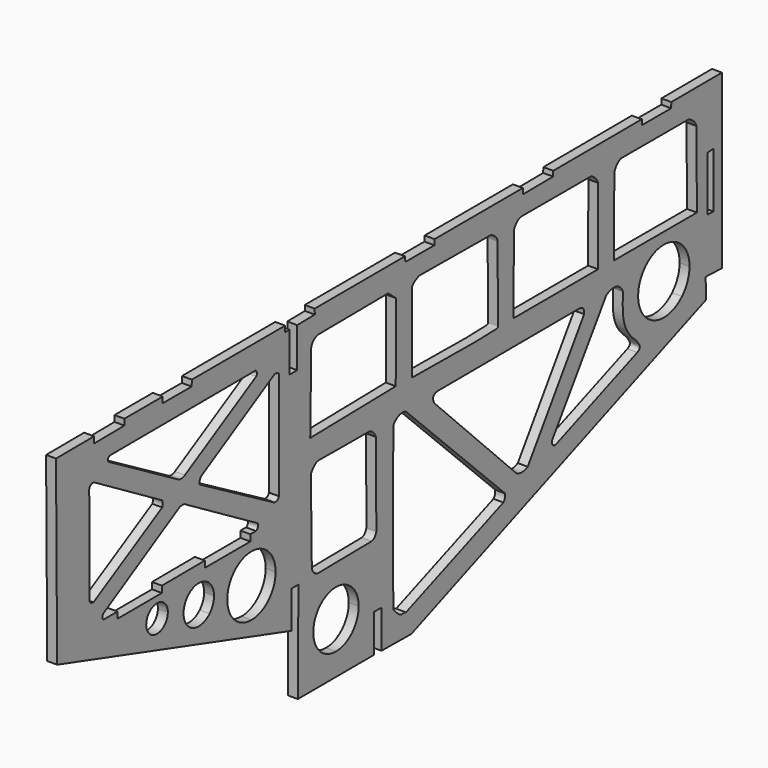
from build123d import *

# Parameters (mm, degrees)
F1_DEPTH = 4


# Not quite as in the source:
# - ends of sketch curves that miss each other by under 0.0002 mm in the source are joined
# - the dataset's text gives a spline's control points without its knots; the knots are read off the source's solid


with BuildPart() as f1:
    # F0 (on Right) → F1 (new body)
    with BuildSketch(Plane.YZ):
        Polygon((-148.644908, 67.35988), (-167.821425, 67.256855), (-167.254463, -6.165021), (-49.042065, -42.167249), (-49.042065, -27.142701), (-45.640268, -27.142701), (-45.92376, -67.680652), (-7.626045, -67.593697), (-7.48542, -52.325631), (-3.764723, -52.349332), (-3.768473, -67.675754), (11.266275, -67.823819), (159.883927, -9.566811), (159.600457, -1.345829), (167.821425, -1.629314), (167.821425, 67.823819), (142.301062, 67.735915), (142.250812, 65.543531), (127.61667, 65.559821), (127.418092, 67.684651), (82.819147, 67.531032), (82.71993, 65.492416), (67.440277, 65.375344), (67.489702, 67.653501), (22.990132, 67.577961), (22.89126, 65.441222), (8.256105, 65.473059), (8.057925, 67.552611), (-37.434053, 67.475386), (-37.384478, 65.338883), (-46.26441, 65.212072), (-46.264583, 49.200648), (-50.03556, 49.197423), (-50.059785, 65.157835), (-52.316775, 65.125607), (-52.316918, 67.503332), (-99.3465, 67.434865), (-99.445935, 65.001045), (-114.179535, 65.035484), (-114.030848, 67.413485), (-133.350465, 67.38536), (-133.37844, 64.951643), (-148.658258, 64.782237), align=None)
        with BuildLine():
            add(Edge.make_bspline(
                [(-18.620168, -39.073955), (-16.475133, -41.218991), (-15.270066, -44.128283), (-15.270067, -47.161822)],
                knots=[0, 0, 0, 0, 1, 1, 1, 1], degree=3))
            add(Edge.make_bspline(
                [(-15.270067, -47.161822), (-15.270069, -53.478835), (-20.391019, -58.599785), (-26.708033, -58.599787)],
                knots=[0, 0, 0, 0, 1, 1, 1, 1], degree=3))
            add(Edge.make_bspline(
                [(-26.708033, -58.599787), (-33.025046, -58.599785), (-38.145996, -53.478835), (-38.145998, -47.161821)],
                knots=[0, 0, 0, 0, 1, 1, 1, 1], degree=3))
            add(Edge.make_bspline(
                [(-38.145998, -47.161821), (-38.145999, -44.128283), (-36.940932, -41.218991), (-34.795897, -39.073955)],
                knots=[0, 0, 0, 0, 1, 1, 1, 1], degree=3))
            add(Edge.make_bspline(
                [(-34.795897, -39.073955), (-32.650862, -36.928919), (-29.741571, -35.72385), (-26.708033, -35.723849)],
                knots=[0, 0, 0, 0, 1, 1, 1, 1], degree=3))
            add(Edge.make_bspline(
                [(-26.708033, -35.723849), (-23.674494, -35.72385), (-20.765203, -36.928919), (-18.620168, -39.073955)],
                knots=[0, 0, 0, 0, 1, 1, 1, 1], degree=3))
        make_face(mode=Mode.SUBTRACT)
        with BuildLine():
            add(Edge.make_bspline(
                [(-116.897902, -4.781812), (-113.891735, -4.781812), (-111.454756, -7.218792), (-111.454755, -10.224959)],
                knots=[0, 0, 0, 0, 1, 1, 1, 1], degree=3))
            add(Edge.make_bspline(
                [(-111.454755, -10.224959), (-111.454756, -13.231126), (-113.891735, -15.668106), (-116.897902, -15.668106)],
                knots=[0, 0, 0, 0, 1, 1, 1, 1], degree=3))
            add(Edge.make_bspline(
                [(-116.897902, -15.668106), (-119.90407, -15.668106), (-122.341049, -13.231126), (-122.34105, -10.224959)],
                knots=[0, 0, 0, 0, 1, 1, 1, 1], degree=3))
            add(Edge.make_bspline(
                [(-122.34105, -10.224959), (-122.341049, -7.218792), (-119.90407, -4.781812), (-116.897902, -4.781812)],
                knots=[0, 0, 0, 0, 1, 1, 1, 1], degree=3))
        make_face(mode=Mode.SUBTRACT)
        with BuildLine():
            add(Edge.make_bspline(
                [(-90.414146, -8.436888), (-88.973656, -9.877378), (-88.164397, -11.831103), (-88.164398, -13.868264)],
                knots=[0, 0, 0, 0, 1, 1, 1, 1], degree=3))
            add(Edge.make_bspline(
                [(-88.164398, -13.868264), (-88.164397, -15.905425), (-88.973656, -17.85915), (-90.414146, -19.29964)],
                knots=[0, 0, 0, 0, 1, 1, 1, 1], degree=3))
            add(Edge.make_bspline(
                [(-90.414146, -19.29964), (-91.854637, -20.74013), (-93.808361, -21.549389), (-95.845522, -21.549389)],
                knots=[0, 0, 0, 0, 1, 1, 1, 1], degree=3))
            add(Edge.make_bspline(
                [(-95.845522, -21.549389), (-97.882684, -21.549389), (-99.836408, -20.74013), (-101.276899, -19.29964)],
                knots=[0, 0, 0, 0, 1, 1, 1, 1], degree=3))
            add(Edge.make_bspline(
                [(-101.276899, -19.29964), (-102.717389, -17.85915), (-103.526648, -15.905425), (-103.526647, -13.868264)],
                knots=[0, 0, 0, 0, 1, 1, 1, 1], degree=3))
            add(Edge.make_bspline(
                [(-103.526647, -13.868264), (-103.526648, -11.831103), (-102.717389, -9.877378), (-101.276899, -8.436888)],
                knots=[0, 0, 0, 0, 1, 1, 1, 1], degree=3))
            add(Edge.make_bspline(
                [(-101.276899, -8.436888), (-99.836408, -6.996398), (-97.882684, -6.187139), (-95.845522, -6.187139)],
                knots=[0, 0, 0, 0, 1, 1, 1, 1], degree=3))
            add(Edge.make_bspline(
                [(-95.845522, -6.187139), (-93.808361, -6.187139), (-91.854637, -6.996398), (-90.414146, -8.436888)],
                knots=[0, 0, 0, 0, 1, 1, 1, 1], degree=3))
        make_face(mode=Mode.SUBTRACT)
        with BuildLine():
            add(Edge.make_bspline(
                [(-69.315802, -5.746334), (-62.588301, -5.746336), (-57.134585, -11.200055), (-57.134587, -17.927556)],
                knots=[0, 0, 0, 0, 1, 1, 1, 1], degree=3))
            add(Edge.make_bspline(
                [(-57.134587, -17.927556), (-57.13459, -24.655055), (-62.588304, -30.108769), (-69.315802, -30.108772)],
                knots=[0, 0, 0, 0, 1, 1, 1, 1], degree=3))
            add(Edge.make_bspline(
                [(-69.315802, -30.108772), (-72.546463, -30.108772), (-75.644804, -28.825399), (-77.929226, -26.540978)],
                knots=[0, 0, 0, 0, 1, 1, 1, 1], degree=3))
            add(Edge.make_bspline(
                [(-77.929226, -26.540978), (-80.213648, -24.256557), (-81.497024, -21.158217), (-81.497025, -17.927556)],
                knots=[0, 0, 0, 0, 1, 1, 1, 1], degree=3))
            add(Edge.make_bspline(
                [(-81.497025, -17.927556), (-81.497026, -14.696895), (-80.213651, -11.598553), (-77.929229, -9.31413)],
                knots=[0, 0, 0, 0, 1, 1, 1, 1], degree=3))
            add(Edge.make_bspline(
                [(-77.929229, -9.31413), (-75.644806, -7.029708), (-72.546464, -5.746333), (-69.315802, -5.746334)],
                knots=[0, 0, 0, 0, 1, 1, 1, 1], degree=3))
        make_face(mode=Mode.SUBTRACT)
        with BuildLine():
            add(Edge.make_bspline(
                [(-39.351915, 9.671161), (-38.178172, 11.208728), (-37.052513, 12.890551), (-35.336048, 12.799936)],
                knots=[0, 0, 0, 0, 1, 1, 1, 1], degree=3))
            Line((-35.336048, 12.799936), (-9.652778, 12.664456))
            add(Edge.make_bspline(
                [(-9.652778, 12.664456), (-8.65323, 12.036301), (-7.709438, 12.077146), (-6.534263, 9.341453)],
                knots=[0, 0, 0, 0, 1, 1, 1, 1], degree=3))
            Line((-6.534263, 9.341453), (-6.37407, -24.324967))
            add(Edge.make_bspline(
                [(-6.37407, -24.324967), (-6.773033, -25.511579), (-7.38825, -26.516122), (-8.681145, -26.774047)],
                knots=[0, 0, 0, 0, 1, 1, 1, 1], degree=3))
            Line((-8.681145, -26.774047), (-36.171038, -27.131302))
            add(Edge.make_bspline(
                [(-36.171038, -27.131302), (-37.79442, -26.594339), (-38.458403, -25.542592), (-38.875838, -24.358559)],
                knots=[0, 0, 0, 0, 1, 1, 1, 1], degree=3))
            Line((-38.875838, -24.358559), (-39.351915, 9.671161))
        make_face(mode=Mode.SUBTRACT)
        with BuildLine():
            add(Edge.make_bspline(
                [(2.256345, 9.947694), (3.321668, 11.731006), (5.932283, 13.337634), (8.607757, 12.202561)],
                knots=[0, 0, 0, 0, 1, 1, 1, 1], degree=3))
            Line((8.607757, 12.202561), (58.543343, -37.151834))
            add(Edge.make_bspline(
                [(58.543343, -37.151834), (58.450905, -38.105316), (58.63884, -39.058807), (57.668505, -40.012296)],
                knots=[0, 0, 0, 0, 1, 1, 1, 1], degree=3))
            Line((57.668505, -40.012296), (8.580412, -59.048722))
            add(Edge.make_bspline(
                [(8.580412, -59.048722), (6.476258, -57.893691), (7.147597, -61.004932), (2.214802, -55.539344)],
                knots=[0, 0, 0, 0, 1, 1, 1, 1], degree=3))
            Line((2.214802, -55.539344), (1.93848, -21.703477))
            Line((1.93848, -21.703477), (2.256345, 9.947694))
        make_face(mode=Mode.SUBTRACT)
        with BuildLine():
            add(Edge.make_bspline(
                [(22.670625, 9.587184), (21.562492, 12.438121), (22.763543, 12.652554), (24.481208, 13.028521)],
                knots=[0, 0, 0, 0, 1, 1, 1, 1], degree=3))
            Line((24.481208, 13.028521), (95.92323, 13.318748))
            add(Edge.make_bspline(
                [(95.92323, 13.318748), (97.785037, 13.164331), (98.57481, 12.132781), (98.378723, 10.294628)],
                knots=[0, 0, 0, 0, 1, 1, 1, 1], degree=3))
            Line((98.378723, 10.294628), (69.937897, -32.299867))
            add(Edge.make_bspline(
                [(69.937897, -32.299867), (68.135137, -33.184687), (66.258735, -33.504959), (64.176825, -32.249617)],
                knots=[0, 0, 0, 0, 1, 1, 1, 1], degree=3))
            Line((64.176825, -32.249617), (22.670625, 9.587184))
        make_face(mode=Mode.SUBTRACT)
        with BuildLine():
            Line((82.129605, -28.036139), (109.42716, 12.304029))
            add(Edge.make_bspline(
                [(117.89025, 10.372148), (116.33766, 14.663858), (111.61056, 14.092876), (109.42716, 12.304029)],
                knots=[0, 0, 0, 0, 1, 1, 1, 1], degree=3))
            add(Edge.make_bspline(
                [(124.473863, -9.554804), (117.165382, -3.288441), (117.750968, 2.209996), (117.89025, 10.372148)],
                knots=[0, 0, 0, 0, 1, 1, 1, 1], degree=3))
            add(Edge.make_bspline(
                [(125.16447, -14.197462), (127.517475, -13.187992), (126.165472, -11.608056), (124.473863, -9.554804)],
                knots=[0, 0, 0, 0, 1, 1, 1, 1], degree=3))
            Line((125.16447, -14.197462), (83.666798, -30.337574))
            add(Edge.make_bspline(
                [(82.129605, -28.036139), (82.148055, -29.242334), (82.464645, -30.183539), (83.666798, -30.337574)],
                knots=[0, 0, 0, 0, 1, 1, 1, 1], degree=3))
        make_face(mode=Mode.SUBTRACT)
        with BuildLine():
            add(Edge.make_bspline(
                [(-105.612742, 24.621151), (-104.715833, 24.842274), (-103.831897, 25.141208), (-102.807255, 24.595951)],
                knots=[0, 0, 0, 0, 1, 1, 1, 1], degree=3))
            Line((-102.807255, 24.595951), (-66.154912, 2.961751))
            add(Edge.make_bspline(
                [(-66.154912, 2.961751), (-65.760262, 1.593474), (-66.306525, 0.997598), (-67.015815, 0.549271)],
                knots=[0, 0, 0, 0, 1, 1, 1, 1], degree=3))
            Line((-67.015815, 0.549271), (-69.892163, 0.578371))
            Line((-69.892163, 0.578371), (-69.857138, -2.021871))
            Line((-69.857138, -2.021871), (-92.658893, -2.047747))
            Line((-92.658893, -2.047747), (-92.833575, 0.562943))
            Line((-92.833575, 0.562943), (-114.442582, 0.439471))
            Line((-114.442582, 0.439471), (-114.477682, -2.154517))
            Line((-114.477682, -2.154517), (-136.928295, -2.214217))
            Line((-136.928295, -2.214217), (-136.822965, 0.348331))
            Line((-136.822965, 0.348331), (-143.79528, 0.352831))
            add(Edge.make_bspline(
                [(-143.79528, 0.352831), (-144.743677, 1.019244), (-144.503138, 1.764908), (-144.065535, 2.523721)],
                knots=[0, 0, 0, 0, 1, 1, 1, 1], degree=3))
            Line((-144.065535, 2.523721), (-105.612742, 24.621151))
        make_face(mode=Mode.SUBTRACT)
        with BuildLine():
            Line((-150.8556, 9.727456), (-151.076168, 49.677209))
            add(Edge.make_bspline(
                [(-148.805078, 51.108666), (-149.672572, 51.183832), (-150.486765, 50.992506), (-151.076168, 49.677209)],
                knots=[0, 0, 0, 0, 1, 1, 1, 1], degree=3))
            Line((-148.805078, 51.108666), (-114.321892, 30.690923))
            add(Edge.make_bspline(
                [(-114.289343, 28.132081), (-113.80962, 28.938256), (-114.035385, 29.884748), (-114.321892, 30.690923)],
                knots=[0, 0, 0, 0, 1, 1, 1, 1], degree=3))
            Line((-114.289343, 28.132081), (-148.953548, 8.563298))
            add(Edge.make_bspline(
                [(-150.8556, 9.727456), (-150.54633, 8.852288), (-149.78526, 8.654813), (-148.953548, 8.563298)],
                knots=[0, 0, 0, 0, 1, 1, 1, 1], degree=3))
        make_face(mode=Mode.SUBTRACT)
        with BuildLine():
            add(Edge.make_bspline(
                [(-95.207468, 28.462321), (-96.091058, 29.456334), (-95.105183, 30.393196), (-94.854623, 31.135171)],
                knots=[0, 0, 0, 0, 1, 1, 1, 1], degree=3))
            Line((-94.854623, 31.135171), (-57.55131, 52.475537))
            add(Edge.make_bspline(
                [(-57.55131, 52.475537), (-56.713065, 52.34595), (-55.721317, 52.561729), (-55.380442, 51.31305)],
                knots=[0, 0, 0, 0, 1, 1, 1, 1], degree=3))
            Line((-55.380442, 51.31305), (-55.436392, 8.191291))
            add(Edge.make_bspline(
                [(-55.436392, 8.191291), (-55.958167, 6.754801), (-56.92437, 6.897586), (-57.81216, 6.925163)],
                knots=[0, 0, 0, 0, 1, 1, 1, 1], degree=3))
            Line((-57.81216, 6.925163), (-95.207468, 28.462321))
        make_face(mode=Mode.SUBTRACT)
        with BuildLine():
            add(Edge.make_bspline(
                [(-141.328215, 55.28627), (-142.026855, 56.205032), (-141.566632, 56.776137), (-140.961495, 57.303767)],
                knots=[0, 0, 0, 0, 1, 1, 1, 1], degree=3))
            Line((-140.961495, 57.303767), (-67.106062, 57.618462))
            add(Edge.make_bspline(
                [(-67.106062, 57.618462), (-66.581768, 56.918597), (-66.11523, 56.212955), (-66.88755, 55.383428)],
                knots=[0, 0, 0, 0, 1, 1, 1, 1], degree=3))
            Line((-66.88755, 55.383428), (-102.865837, 34.965384))
            add(Edge.make_bspline(
                [(-102.865837, 34.965384), (-103.758585, 34.340003), (-105.563392, 34.272698), (-106.45614, 34.954958)],
                knots=[0, 0, 0, 0, 1, 1, 1, 1], degree=3))
            Line((-106.45614, 34.954958), (-141.328215, 55.28627))
        make_face(mode=Mode.SUBTRACT)
        with BuildLine():
            Line((3.40464, 23.317126), (-39.681795, 22.478071))
            Line((-39.681795, 22.478071), (-39.16287, 54.705703))
            add(Edge.make_bspline(
                [(-35.542463, 57.545455), (-38.127855, 56.943518), (-38.642985, 55.824017), (-39.16287, 54.705703)],
                knots=[0, 0, 0, 0, 1, 1, 1, 1], degree=3))
            Line((-35.542463, 57.545455), (-0.401647, 57.864805))
            Line((-0.401647, 57.864805), (3.61512, 54.464192))
            Line((3.61512, 54.464192), (3.40464, 23.317126))
        make_face(mode=Mode.SUBTRACT)
        with BuildLine():
            add(Edge.make_bspline(
                [(147.694844, 14.847532), (150.122505, 12.419871), (151.486351, 9.127255), (151.48635, 5.694024)],
                knots=[0, 0, 0, 0, 1, 1, 1, 1], degree=3))
            add(Edge.make_bspline(
                [(151.48635, 5.694024), (151.486351, 2.260792), (150.122505, -1.031824), (147.694844, -3.459485)],
                knots=[0, 0, 0, 0, 1, 1, 1, 1], degree=3))
            add(Edge.make_bspline(
                [(147.694844, -3.459485), (145.267182, -5.887146), (141.974567, -7.250992), (138.541335, -7.250992)],
                knots=[0, 0, 0, 0, 1, 1, 1, 1], degree=3))
            add(Edge.make_bspline(
                [(138.541335, -7.250992), (135.108103, -7.250992), (131.815488, -5.887146), (129.387826, -3.459485)],
                knots=[0, 0, 0, 0, 1, 1, 1, 1], degree=3))
            add(Edge.make_bspline(
                [(129.387826, -3.459485), (126.960165, -1.031824), (125.596319, 2.260792), (125.59632, 5.694024)],
                knots=[0, 0, 0, 0, 1, 1, 1, 1], degree=3))
            add(Edge.make_bspline(
                [(125.59632, 5.694024), (125.596319, 9.127255), (126.960165, 12.419871), (129.387826, 14.847532)],
                knots=[0, 0, 0, 0, 1, 1, 1, 1], degree=3))
            add(Edge.make_bspline(
                [(129.387826, 14.847532), (131.815488, 17.275193), (135.108103, 18.639039), (138.541335, 18.639039)],
                knots=[0, 0, 0, 0, 1, 1, 1, 1], degree=3))
            add(Edge.make_bspline(
                [(138.541335, 18.639039), (141.974567, 18.639039), (145.267182, 17.275193), (147.694844, 14.847532)],
                knots=[0, 0, 0, 0, 1, 1, 1, 1], degree=3))
        make_face(mode=Mode.SUBTRACT)
        Polygon((160.453747, 20.333258), (160.442348, 42.316125), (163.633642, 42.5266), (163.504733, 20.266134), align=None, mode=Mode.SUBTRACT)
        with BuildLine():
            Line((11.625622, 23.036491), (11.496892, 54.634844))
            add(Edge.make_bspline(
                [(15.063375, 57.758778), (13.2666, 56.920116), (11.635665, 56.026175), (11.496892, 54.634844)],
                knots=[0, 0, 0, 0, 1, 1, 1, 1], degree=3))
            Line((15.063375, 57.758778), (51.656947, 57.497084))
            add(Edge.make_bspline(
                [(54.7035, 53.967384), (54.608355, 55.669877), (52.999043, 56.507134), (51.656947, 57.497084)],
                knots=[0, 0, 0, 0, 1, 1, 1, 1], degree=3))
            add(Edge.make_bspline(
                [(54.995535, 23.317126), (54.995535, 24.4421922109), (54.7072906561, 53.5842116305), (54.7035118829, 53.9661829773), (54.703511821, 53.9661891125), (54.7035, 53.967384)],
                knots=[0, 0, 0, 0, 0.9921875, 0.9947916667, 1, 1, 1, 1], degree=3))
            add(Edge.make_bspline(
                [(11.625622, 23.036491), (11.627377535, 23.0364565802), (11.6273867263, 23.0364562793), (12.1885696826, 23.0254612225), (54.995535, 22.1920528438), (54.995535, 23.317126)],
                knots=[0, 0, 0, 0, 0.0052083333, 0.0078125, 1, 1, 1, 1], degree=3))
        make_face(mode=Mode.SUBTRACT)
        with BuildLine():
            Line((62.806965, 23.322826), (62.958585, 54.565879))
            add(Edge.make_bspline(
                [(66.654277, 57.834636), (64.46103, 57.345894), (63.68658, 55.970402), (62.958585, 54.565879)],
                knots=[0, 0, 0, 0, 1, 1, 1, 1], degree=3))
            Line((66.654277, 57.834636), (102.033803, 57.817546))
            add(Edge.make_bspline(
                [(105.487935, 53.975549), (104.430863, 56.482164), (103.216073, 56.938433), (102.033803, 57.817546)],
                knots=[0, 0, 0, 0, 1, 1, 1, 1], degree=3))
            Line((105.487935, 53.975549), (105.379507, 23.390101))
            Line((105.379507, 23.390101), (62.806965, 23.322826))
        make_face(mode=Mode.SUBTRACT)
        with BuildLine():
            add(Edge.make_bspline(
                [(113.594888, 54.452726), (114.097598, 55.917625), (115.05702, 57.263287), (117.005655, 58.050776)],
                knots=[0, 0, 0, 0, 1, 1, 1, 1], degree=3))
            Line((117.005655, 58.050776), (151.011975, 58.042412))
            add(Edge.make_bspline(
                [(151.011975, 58.042412), (152.69778, 57.301999), (154.428885, 56.060678), (154.99173, 54.065194)],
                knots=[0, 0, 0, 0, 1, 1, 1, 1], degree=3))
            Line((154.99173, 54.065194), (155.210752, 23.252665))
            Line((155.210752, 23.252665), (113.395703, 23.249665))
            Line((113.395703, 23.249665), (113.594888, 54.452726))
        make_face(mode=Mode.SUBTRACT)
    extrude(amount=F1_DEPTH)


solid = f1.part
